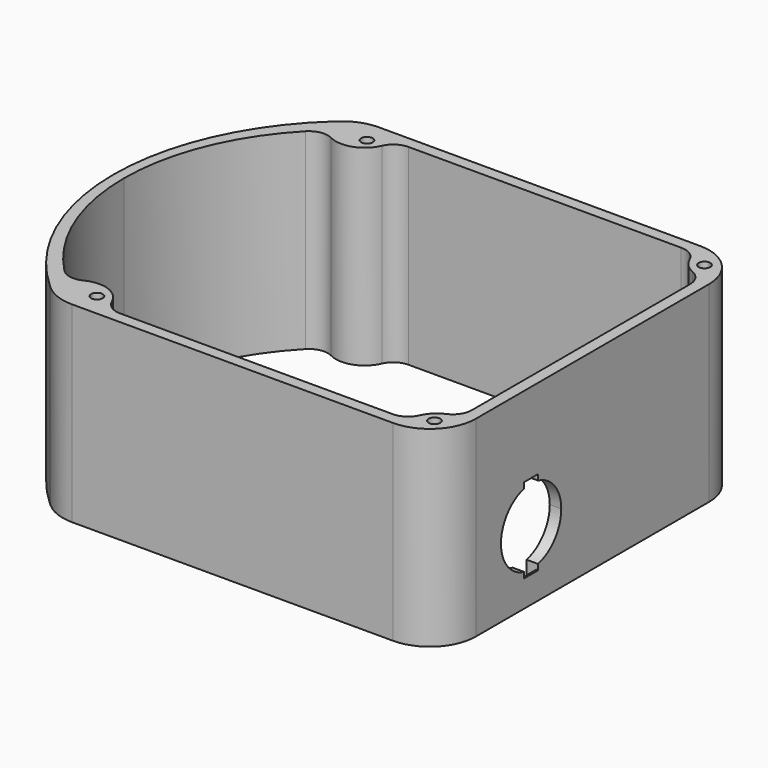
from build123d import *

# Parameters (mm, degrees)
F0_R     = 1.5
F1_DEPTH = 50
F2_R     = 12
F3_R     = 5
F5_DEPTH = 4
F6_SIZE  = 2.5


with BuildPart() as f1:
    # F0 (on Top) → F1 (new body)
    with BuildSketch(Plane.XY):
        with BuildLine():
            Line((40.1261364576, -50), (50, -50))
            Line((50, -50), (50, -40.1261364576))
            ThreePointArc((50, -40.1261364576), (48.5323223277, -39.658202653), (47, -39.5))
            Line((47, -39.5), (47, -47))
            Line((47, -47), (39.5, -47))
            ThreePointArc((39.5, -47), (39.658202653, -48.5323223277), (40.1261364576, -50))
        make_face()
        with BuildLine():
            Line((-40.1261364576, -50), (40.1261364576, -50))
            ThreePointArc((40.1261364576, -50), (39.658202653, -48.5323223277), (39.5, -47))
            Line((39.5, -47), (-39.5, -47))
            ThreePointArc((-39.5, -47), (-39.658202653, -48.5323223277), (-40.1261364576, -50))
        make_face()
        with BuildLine():
            ThreePointArc((47, -39.5), (48.5323223277, -39.658202653), (50, -40.1261364576))
            Line((50, -40.1261364576), (50, 40.1261364576))
            ThreePointArc((50, 40.1261364576), (48.5323223277, 39.658202653), (47, 39.5))
            Line((47, 39.5), (47, -39.5))
        make_face()
        with BuildLine():
            Line((-50, -50), (-40.1261364576, -50))
            ThreePointArc((-40.1261364576, -50), (-39.658202653, -48.5323223277), (-39.5, -47))
            Line((-39.5, -47), (-44, -47))
            Line((-44, -47), (-47, -47))
            ThreePointArc((-47, -47), (-50.0530276117, -44.8189291928), (-52.9544285232, -42.4398705103))
            ThreePointArc((-52.9544285232, -42.4398705103), (-53.9803824114, -44.2569612852), (-54.4659740059, -46.2863949669))
            ThreePointArc((-54.4659740059, -46.2863949669), (-52.2760251532, -48.1949550771), (-50, -50))
        make_face()
        with BuildLine():
            ThreePointArc((47, -39.5), (41.6966991411, -41.6966991411), (39.5, -47))
            Line((39.5, -47), (47, -47))
            Line((47, -47), (47, -39.5))
        make_face()
        with Locations((44, -44)):
            Circle(F0_R, mode=Mode.SUBTRACT)
        with BuildLine():
            ThreePointArc((47, 39.5), (48.5323223277, 39.658202653), (50, 40.1261364576))
            Line((50, 40.1261364576), (50, 50))
            Line((50, 50), (40.1261364576, 50))
            ThreePointArc((40.1261364576, 50), (39.658202653, 48.5323223277), (39.5, 47))
            Line((39.5, 47), (44, 47))
            Line((44, 47), (47, 47))
            Line((47, 47), (47, 44))
            Line((47, 44), (47, 39.5))
        make_face()
        with BuildLine():
            ThreePointArc((-54.4659740059, 46.2863949669), (-74.8805891399, 0), (-54.4659740059, -46.2863949669))
            ThreePointArc((-54.4659740059, -46.2863949669), (-53.9803824114, -44.2569612852), (-52.9544285232, -42.4398705103))
            ThreePointArc((-52.9544285232, -42.4398705103), (-67.1504896249, -23.2960258249), (-72.1814061329, 0))
            ThreePointArc((-72.1814061329, 0), (-67.1504896249, 23.2960258249), (-52.9544285232, 42.4398705103))
            ThreePointArc((-52.9544285232, 42.4398705103), (-53.9803824114, 44.2569612852), (-54.4659740059, 46.2863949669))
        make_face()
        with BuildLine():
            Line((-44, -47), (-39.5, -47))
            ThreePointArc((-39.5, -47), (-44.5925338968, -39.8968945551), (-52.9544285232, -42.4398705103))
            ThreePointArc((-52.9544285232, -42.4398705103), (-50.0530276117, -44.8189291928), (-47, -47))
            Line((-47, -47), (-44, -47))
        make_face()
        with BuildLine():
            ThreePointArc((-42.5, -44), (-42.9393398282, -45.0606601718), (-44, -45.5))
            ThreePointArc((-44, -45.5), (-45.0606601718, -45.0606601718), (-45.5, -44))
            ThreePointArc((-45.5, -44), (-44, -42.5), (-42.5, -44))
        make_face(mode=Mode.SUBTRACT)
        with BuildLine():
            ThreePointArc((39.5, 47), (41.6966991411, 41.6966991411), (47, 39.5))
            Line((47, 39.5), (47, 44))
            Line((47, 44), (45.5, 44))
            ThreePointArc((45.5, 44), (42.9393398282, 42.9393398282), (44, 45.5))
            Line((44, 45.5), (44, 47))
            Line((44, 47), (39.5, 47))
        make_face()
        with BuildLine():
            ThreePointArc((-50, 50), (-52.2760251532, 48.1949550771), (-54.4659740059, 46.2863949669))
            ThreePointArc((-54.4659740059, 46.2863949669), (-53.9803824114, 44.2569612852), (-52.9544285232, 42.4398705103))
            ThreePointArc((-52.9544285232, 42.4398705103), (-50.0530276117, 44.8189291928), (-47, 47))
            Line((-47, 47), (-39.5, 47))
            ThreePointArc((-39.5, 47), (-39.658202653, 48.5323223277), (-40.1261364576, 50))
            Line((-40.1261364576, 50), (-50, 50))
        make_face()
        with BuildLine():
            ThreePointArc((39.5, 47), (39.658202653, 48.5323223277), (40.1261364576, 50))
            Line((40.1261364576, 50), (-40.1261364576, 50))
            ThreePointArc((-40.1261364576, 50), (-39.658202653, 48.5323223277), (-39.5, 47))
            Line((-39.5, 47), (39.5, 47))
        make_face()
        with BuildLine():
            Line((45.5, 44), (47, 44))
            Line((47, 44), (47, 47))
            Line((47, 47), (44, 47))
            Line((44, 47), (44, 45.5))
            ThreePointArc((44, 45.5), (45.0606601718, 45.0606601718), (45.5, 44))
        make_face()
        with BuildLine():
            ThreePointArc((-47, 47), (-50.0530276117, 44.8189291928), (-52.9544285232, 42.4398705103))
            ThreePointArc((-52.9544285232, 42.4398705103), (-44.5925338968, 39.8968945551), (-39.5, 47))
            Line((-39.5, 47), (-47, 47))
        make_face()
        with Locations((-44, 44)):
            Circle(F0_R, mode=Mode.SUBTRACT)
    extrude(amount=F1_DEPTH)

    # F2
    f2_edges = [f1.edges().sort_by_distance(p)[0] for p in [
        (-50, 50, 25),
        (50, 50, 25),
        (50, -50, 25),
        (-50, -50, 25),
    ]]
    fillet(f2_edges, radius=F2_R)

    # F3
    f3_edges = [f1.edges().sort_by_distance(p)[0] for p in [
        (-39.5, -47, 25),
        (39.5, -47, 25),
        (47, -39.5, 25),
        (39.5, 47, 25),
        (47, 39.5, 25),
        (-39.5, 47, 25),
        (-52.954429, -42.439871, 25),
        (-52.954429, 42.439871, 25),
    ]]
    fillet(f3_edges, radius=F3_R)

    # F4 (on face) → F5 (cut)
    with BuildSketch(Plane.YZ.offset(50)):
        with BuildLine():
            Line((-22.25, 8.4361030432), (-22.25, 27.5638969568))
            ThreePointArc((-22.25, 27.5638969568), (-29.825, 18), (-22.25, 8.4361030432))
        make_face()
        with BuildLine():
            Line((-17.75, 8.4361030432), (-17.75, 27.5638969568))
            ThreePointArc((-17.75, 27.5638969568), (-20, 27.825), (-22.25, 27.5638969568))
            Line((-22.25, 27.5638969568), (-22.25, 8.4361030432))
            ThreePointArc((-22.25, 8.4361030432), (-20, 8.175), (-17.75, 8.4361030432))
        make_face()
        with BuildLine():
            ThreePointArc((-17.75, 8.4361030432), (-12.2981536305, 11.8998206994), (-10.175, 18))
            ThreePointArc((-10.175, 18), (-12.2981536305, 24.1001793006), (-17.75, 27.5638969568))
            Line((-17.75, 27.5638969568), (-17.75, 8.4361030432))
        make_face()
        with BuildLine():
            ThreePointArc((-22.25, 27.5638969568), (-20, 27.825), (-17.75, 27.5638969568))
            Line((-17.75, 27.5638969568), (-17.75, 29.05))
            Line((-17.75, 29.05), (-22.25, 29.05))
            Line((-22.25, 29.05), (-22.25, 27.5638969568))
        make_face()
        with BuildLine():
            Line((-17.75, 6.95), (-17.75, 8.4361030432))
            ThreePointArc((-17.75, 8.4361030432), (-20, 8.175), (-22.25, 8.4361030432))
            Line((-22.25, 8.4361030432), (-22.25, 6.95))
            Line((-22.25, 6.95), (-17.75, 6.95))
        make_face()
    extrude(amount=-F5_DEPTH, mode=Mode.SUBTRACT)

    # F6
    f6_edges = [f1.edges().sort_by_distance(p)[0] for p in [
        (47, -20, 29.05),
        (47, -20, 6.95),
    ]]
    chamfer(f6_edges, length=F6_SIZE)


solid = f1.part
